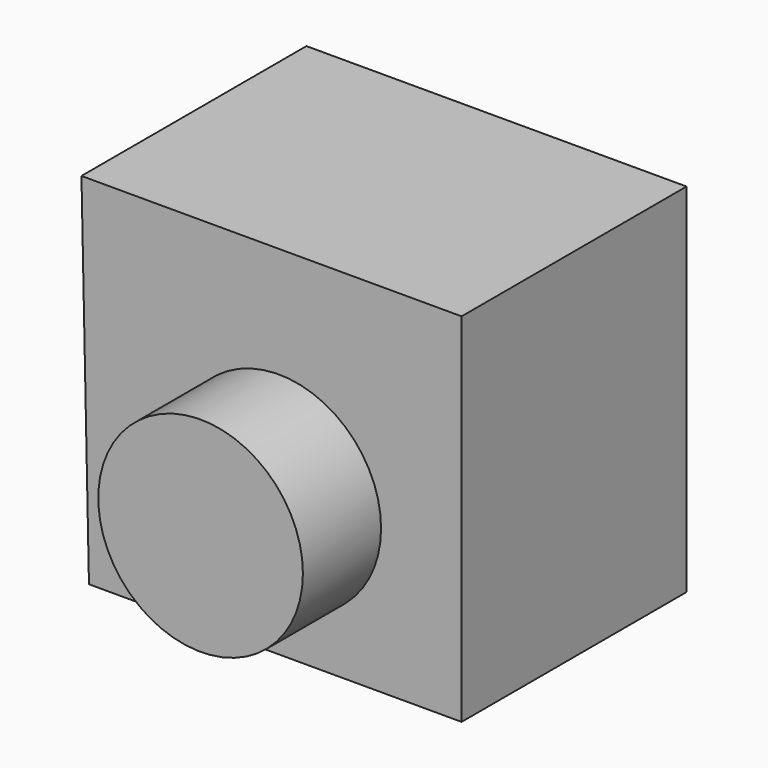
from build123d import *

# Parameters (mm, degrees)
F1_DEPTH = 73.1121525168
F2_R     = 26.6044020107
F3_DEPTH = 25.4


# Not quite as in the source:
# - the program builds the solid bodies; features that only make, move or delete a surface that nothing else refers to are left out


with BuildPart() as f1:
    # F0 (on Front) → F1 (new body)
    with BuildSketch(Plane.XZ):
        Polygon((-51.2930899858, 55.3425773978), (-49.3433475494, -37.4949574471), (47.5436300039, -37.4949574471), (47.5436300039, 55.3425773978), align=None)
    extrude(amount=F1_DEPTH)

    # F2 (on face) → F3 (join)
    with BuildSketch(Plane.XZ.offset(73.1121525168)):
        Circle(F2_R)
    extrude(amount=F3_DEPTH)


solid = f1.part
